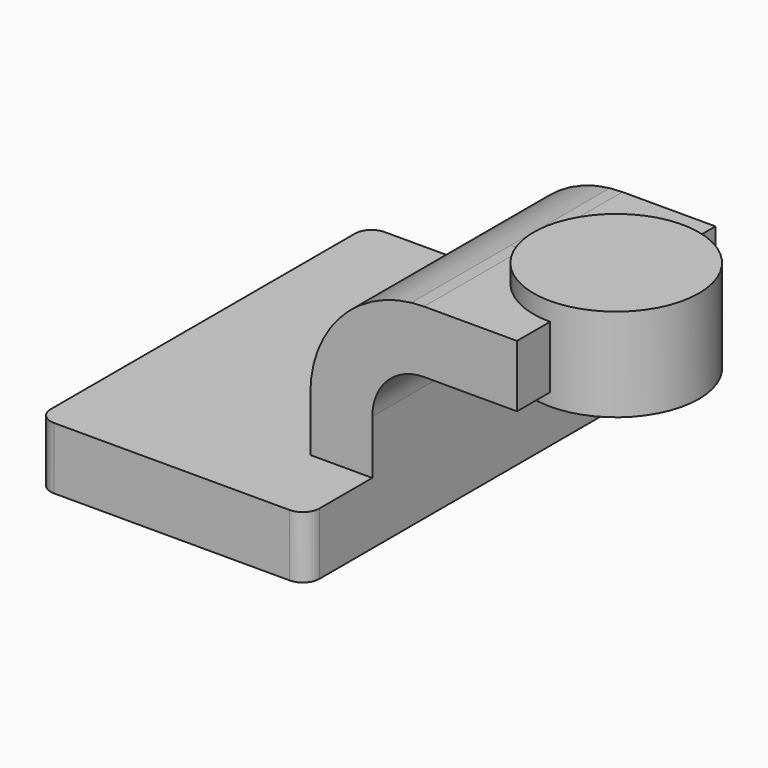
from build123d import *

# Parameters (mm, degrees)
F1_DEPTH = 63.5
F2_DEPTH = 38.1
F4_R     = 5.08
F5_R     = 5.08


with BuildPart() as f1:
    # F0 (on Front) → F1 (new body, symmetric)
    with BuildSketch(Plane.XZ):
        Polygon((-41.275, -9.525), (41.275, -9.525), (41.275, 9.525), (22.225, 9.525), (-41.275, 9.525), align=None)
    extrude(amount=F1_DEPTH, both=True)

    # F0 (on Front) → F2 (join, symmetric)
    with BuildSketch(Plane.XZ):
        with BuildLine():
            Line((22.225, 9.525), (41.275, 9.525))
            Line((41.275, 9.525), (41.275, 26.1178162626))
            ThreePointArc((41.275, 26.1178162626), (45.9246798487, 37.3431364139), (57.15, 41.9928162626))
            Line((57.15, 41.9928162626), (60.325, 41.9928162626))
            Line((60.325, 41.9928162626), (60.325, 61.0428162626))
            Line((60.325, 61.0428162626), (57.15, 61.0428162626))
            add(Edge.make_bspline(
                [(53.270143605, 60.8266384747), (54.5515105063, 60.9068312899), (55.8448088672, 60.9788851621), (57.15, 61.0428162626)],
                knots=[108.4277797835, 108.4277797835, 108.4277797835, 108.4277797835, 111.0926010924, 111.0926010924, 111.0926010924, 111.0926010924], degree=3))
            ThreePointArc((53.270143605, 60.8266384747), (31.1186764686, 49.4014117796), (22.225, 26.1178162626))
            Line((22.225, 26.1178162626), (22.225, 9.525))
        make_face()
        Polygon((60.325, 61.0428162626), (60.325, 41.9928162626), (60.325, 41.9873446226), (85.725, 41.9873446226), (85.725, 42.3024737561), (85.725, 51.9704466166), (85.725, 52.3875), (85.725, 61.0428162626), align=None)
    extrude(amount=F2_DEPTH, both=True)

    # F0 (on Front) → F3 (revolve)
    with BuildSketch(Plane.XZ):
        Polygon((85.725, 66.675), (85.725, 61.0428162626), (85.725, 52.3875), (85.725, 51.9704466166), (85.725, 42.3024737561), (85.725, 41.9873446226), (85.725, 38.1), (111.125, 38.1), (111.125, 66.675), align=None)
    revolve(axis=Axis((85.725, 0, 56.7151581313), (0, 0, -1)))

    # F4
    f4_edges = [f1.edges().sort_by_distance(p)[0] for p in [
        (41.275, -63.5, 0),
    ]]
    fillet(f4_edges, radius=F4_R)

    # F5
    f5_edges = [f1.edges().sort_by_distance(p)[0] for p in [
        (-41.275, 63.5, 0),
        (-41.275, -63.5, 0),
        (41.275, 63.5, 0),
    ]]
    fillet(f5_edges, radius=F5_R)


solid = f1.part
